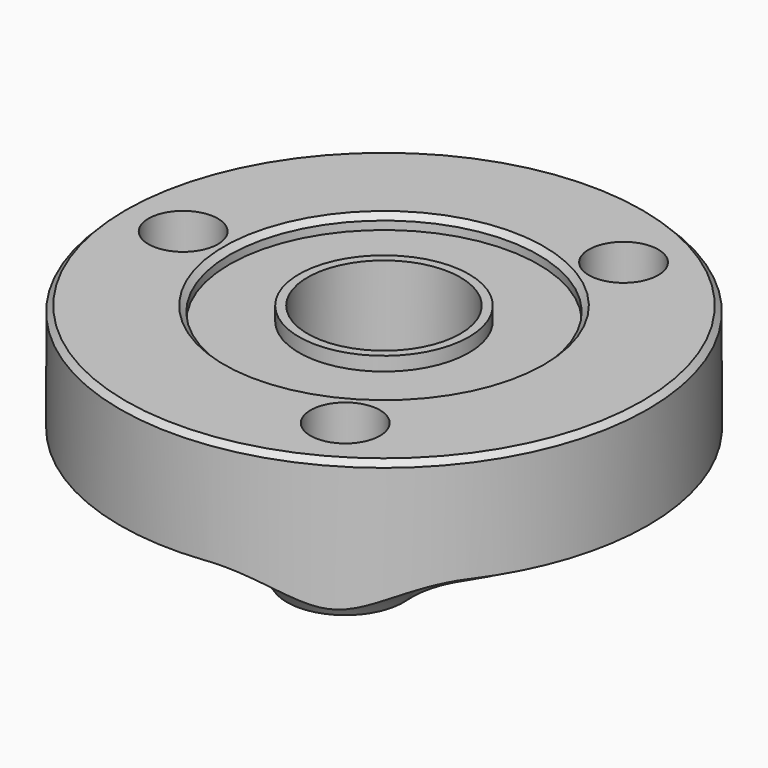
from build123d import *

# Parameters (mm, degrees)
F0_R         = 12.065
F0_R_2       = 1.5875
F0_R_3       = 3.8862
F0_R_4       = 3.4925
F1_DEPTH     = 6.35
F2_R         = 7.0612
F2_R_2       = 3.8862
F3_DEPTH     = 0.635
F4_SIZE      = 0.254
F5_R         = 12.065
F6_DEPTH     = 1.4224
F7_T2_ANGLE  = 68.0844261326
F7_T6_ANGLE  = 38.3538722805
F7_S7_R      = 12.065
F7_T8_DEPTH  = 3
F7_T12_ANGLE = 128.6233184284
F7_S13_R     = 12.065
F7_T14_DEPTH = 7
F7_T18_ANGLE = 38.3538722805
F7_S19_R     = 12.065
F7_T20_DEPTH = 3
F7_T24_ANGLE = 128.6233184284
F7_S25_R     = 12.065
F7_T26_DEPTH = 9
F7_T28_ANGLE = 68.0844261326
F7_T32_ANGLE = 38.3538722805
F7_S33_R     = 12.065
F7_T34_DEPTH = 3
F7_T38_ANGLE = 38.3538722805
F7_S39_R     = 12.065
F7_T40_DEPTH = 3
F7_T42_ANGLE = 68.0844261326
F7_T46_ANGLE = 38.3538722805
F7_S47_R     = 12.065
F7_T48_DEPTH = 4
F7_T52_ANGLE = 128.6233184284
F7_S53_R     = 12.065
F7_T54_DEPTH = 7
F7_T58_ANGLE = 38.3538722805
F7_S59_R     = 12.065
F7_T60_DEPTH = 4


# Not quite as in the source:
# - a fillet or chamfer that OpenCascade refuses, or shapes differently, is made with other operations: its cross-section is extruded or revolved along the edge and cut away or added


with BuildPart() as f1:
    # F0 (on Top) → F1 (new body)
    with BuildSketch(Plane.XY):
        Circle(F0_R)
        with Locations((4.59105, -7.9519318601)):
            Circle(F0_R_2, mode=Mode.SUBTRACT)
        with Locations((-9.1821, 0)):
            Circle(F0_R_2, mode=Mode.SUBTRACT)
        Circle(F0_R_3, mode=Mode.SUBTRACT)
        with Locations((4.59105, 7.9519318601)):
            Circle(F0_R_2, mode=Mode.SUBTRACT)
        Circle(F0_R_3)
        Circle(F0_R_4, mode=Mode.SUBTRACT)
    extrude(amount=F1_DEPTH)

    # F2 (on face) → F3 (cut)
    with BuildSketch(Plane.XY.offset(6.35)):
        Circle(F2_R)
        Circle(F2_R_2, mode=Mode.SUBTRACT)
    extrude(amount=-F3_DEPTH, mode=Mode.SUBTRACT)

    # F4
    f4_edges = [f1.edges().sort_by_distance(p)[0] for p in [
        (-7.0612, 0, 6.35),
        (-12.065, 0, 6.35),
    ]]
    chamfer(f4_edges, length=F4_SIZE)

    # F5 (on face) → F6 (cut)
    with BuildSketch(Plane(origin=(0, 0, 0), x_dir=(1, 0, 0), z_dir=(0, 0, -1))):
        Circle(F5_R)
        with BuildLine():
            ThreePointArc((0.6714307473, -9.5013054762), (-4.7625, -8.248891971), (-8.5640872851, -4.1691766541))
            ThreePointArc((-8.5640872851, -4.1691766541), (-9.3019875524, -3.1364431851), (-10.3381797291, -2.4034077182))
            ThreePointArc((-10.3381797291, -2.4034077182), (-11.8491, 0), (-10.3381797291, 2.4034077182))
            ThreePointArc((-10.3381797291, 2.4034077182), (-9.3019875524, 3.1364431851), (-8.5640872851, 4.1691766541))
            ThreePointArc((-8.5640872851, 4.1691766541), (-4.7625, 8.248891971), (0.6714307473, 9.5013054762))
            ThreePointArc((0.6714307473, 9.5013054762), (1.9347543004, 9.6239791186), (3.0876777249, 10.1548301334))
            ThreePointArc((3.0876777249, 10.1548301334), (5.92455, 10.261621612), (7.2505020042, 7.7514224152))
            ThreePointArc((7.2505020042, 7.7514224152), (7.367233252, 6.4875359336), (7.8926565378, 5.3321288221))
            ThreePointArc((7.8926565378, 5.3321288221), (9.525, 0), (7.8926565378, -5.3321288221))
            ThreePointArc((7.8926565378, -5.3321288221), (7.367233252, -6.4875359336), (7.2505020042, -7.7514224152))
            ThreePointArc((7.2505020042, -7.7514224152), (5.92455, -10.261621612), (3.0876777249, -10.1548301334))
            ThreePointArc((3.0876777249, -10.1548301334), (1.9347543004, -9.6239791186), (0.6714307473, -9.5013054762))
        make_face(mode=Mode.SUBTRACT)
    extrude(amount=-F6_DEPTH, mode=Mode.SUBTRACT)

    # F7: fillet of radius 2.794 on 11 edges, made by hand

    # F7_s1 → F7_t2 (revolve)
    with BuildSketch(Plane(origin=(0, 0, 0), x_dir=(0, 0, 1), z_dir=(-0.5598035509, -0.8286253583, 0))):
        with BuildLine():
            ThreePointArc((1.4224, -11.9591629855), (1.0407314863, -10.5495201939), (0, -9.525))
            Line((0, -9.525), (1.4224, -9.525))
            Line((1.4224, -9.525), (1.4224, -11.9591629855))
        make_face()
    revolve(axis=Axis((0, 0, 1.4224), (0, 0, 1)), revolution_arc=F7_T2_ANGLE)


with BuildPart() as f7_tool4:
    # F7_s5 → F7_t6 (revolve)
    with BuildSketch(Plane(origin=(0, 0, 0), x_dir=(0, 0, 1), z_dir=(0.5598035509, -0.8286253583, 0))):
        with BuildLine():
            ThreePointArc((1.4224, -11.9591629855), (1.0407314863, -10.5495201939), (0, -9.525))
            Line((0, -9.525), (1.4224, -9.525))
            Line((1.4224, -9.525), (1.4224, -11.9591629855))
        make_face()
    revolve(axis=Axis((11.049719153, 7.464980351, 1.4224), (0, 0, -1)), revolution_arc=F7_T6_ANGLE)

    # F7_s7 → F7_t8 (intersect, symmetric)
    with BuildSketch(Plane.XY.offset(0.7)):
        Circle(F7_S7_R)
    extrude(amount=F7_T8_DEPTH, both=True, mode=Mode.INTERSECT)


with BuildPart() as f1_1:
    add(f1.part)

    # F7_t3: union F7_tool4
    add(f7_tool4.part)


with BuildPart() as f7_tool10:
    # F7_s11 → F7_t12 (revolve)
    with BuildSketch(Plane(origin=(0.622097238, 8.2511711447, 0), x_dir=(0, 0, 1), z_dir=(-0.0751816441, -0.9971698553, 0))):
        with BuildLine():
            ThreePointArc((1.4224, -9.0813803384), (1.0407314863, -7.6717375468), (0, -6.6472173529))
            Line((0, -6.6472173529), (1.4224, -6.6472173529))
            Line((1.4224, -6.6472173529), (1.4224, -9.0813803384))
        make_face()
    revolve(axis=Axis((4.59105, 7.9519318601, 1.4224), (0, 0, 1)), revolution_arc=F7_T12_ANGLE)

    # F7_s13 → F7_t14 (intersect, symmetric)
    with BuildSketch(Plane.XY):
        Circle(F7_S13_R)
    extrude(amount=F7_T14_DEPTH, both=True, mode=Mode.INTERSECT)


with BuildPart() as f1_2:
    add(f1_1.part)

    # F7_t9: union F7_tool10
    add(f7_tool10.part)


with BuildPart() as f7_tool16:
    # F7_s17 → F7_t18 (revolve)
    with BuildSketch(Plane(origin=(0.622097238, -8.2511711447, 0), x_dir=(0, 0, 1), z_dir=(0.0751816441, -0.9971698553, 0))):
        with BuildLine():
            ThreePointArc((1.4224, -9.0813803384), (1.0407314863, -7.6717375468), (0, -6.6472173529))
            Line((0, -6.6472173529), (1.4224, -6.6472173529))
            Line((1.4224, -6.6472173529), (1.4224, -9.0813803384))
        make_face()
    revolve(axis=Axis((11.049719153, -7.464980351, 1.4224), (0, 0, -1)), revolution_arc=F7_T18_ANGLE)

    # F7_s19 → F7_t20 (intersect, symmetric)
    with BuildSketch(Plane.XY.offset(0.7)):
        Circle(F7_S19_R)
    extrude(amount=F7_T20_DEPTH, both=True, mode=Mode.INTERSECT)


with BuildPart() as f1_3:
    add(f1_2.part)

    # F7_t15: union F7_tool16
    add(f7_tool16.part)


with BuildPart() as f7_tool22:
    # F7_s23 → F7_t24 (revolve)
    with BuildSketch(Plane(origin=(6.8346752033, -4.6643375841, 0), x_dir=(0, 0, 1), z_dir=(-0.8259836045, 0.5636941414, 0))):
        with BuildLine():
            ThreePointArc((1.4224, -9.0813803384), (1.0407314863, -7.6717375468), (0, -6.6472173529))
            Line((0, -6.6472173529), (1.4224, -6.6472173529))
            Line((1.4224, -6.6472173529), (1.4224, -9.0813803384))
        make_face()
    revolve(axis=Axis((4.59105, -7.9519318601, 1.4224), (0, 0, 1)), revolution_arc=F7_T24_ANGLE)

    # F7_s25 → F7_t26 (intersect, symmetric)
    with BuildSketch(Plane.XY):
        Circle(F7_S25_R)
    extrude(amount=F7_T26_DEPTH, both=True, mode=Mode.INTERSECT)


with BuildPart() as f1_4:
    add(f1_3.part)

    # F7_t21: union F7_tool22
    add(f7_tool22.part)

    # F7_s27 → F7_t28 (revolve)
    with BuildSketch(Plane(origin=(0, 0, 0), x_dir=(0, 0, 1), z_dir=(0.997512386, -0.070491417, 0))):
        with BuildLine():
            ThreePointArc((1.4224, -11.9591629855), (1.0407314863, -10.5495201939), (0, -9.525))
            Line((0, -9.525), (1.4224, -9.525))
            Line((1.4224, -9.525), (1.4224, -11.9591629855))
        make_face()
    revolve(axis=Axis((0, 0, 1.4224), (0, 0, 1)), revolution_arc=F7_T28_ANGLE)


with BuildPart() as f7_tool30:
    # F7_s31 → F7_t32 (revolve)
    with BuildSketch(Plane(origin=(6.8346752033, 4.6643375841, 0), x_dir=(0, 0, 1), z_dir=(0.8259836045, 0.5636941414, 0))):
        with BuildLine():
            ThreePointArc((1.4224, -9.0813803384), (1.0407314863, -7.6717375468), (0, -6.6472173529))
            Line((0, -6.6472173529), (1.4224, -6.6472173529))
            Line((1.4224, -6.6472173529), (1.4224, -9.0813803384))
        make_face()
    revolve(axis=Axis((0.9400030462, 13.3018276666, 1.4224), (0, 0, -1)), revolution_arc=F7_T32_ANGLE)

    # F7_s33 → F7_t34 (intersect, symmetric)
    with BuildSketch(Plane.XY.offset(0.7)):
        Circle(F7_S33_R)
    extrude(amount=F7_T34_DEPTH, both=True, mode=Mode.INTERSECT)


with BuildPart() as f1_5:
    add(f1_4.part)

    # F7_t29: union F7_tool30
    add(f7_tool30.part)


with BuildPart() as f7_tool36:
    # F7_s37 → F7_t38 (revolve)
    with BuildSketch(Plane(origin=(0, 0, 0), x_dir=(0, 0, 1), z_dir=(-0.997512386, -0.070491417, 0))):
        with BuildLine():
            ThreePointArc((1.4224, -11.9591629855), (1.0407314863, -10.5495201939), (0, -9.525))
            Line((0, -9.525), (1.4224, -9.525))
            Line((1.4224, -9.525), (1.4224, -11.9591629855))
        make_face()
    revolve(axis=Axis((0.9400030462, -13.3018276666, 1.4224), (0, 0, -1)), revolution_arc=F7_T38_ANGLE)

    # F7_s39 → F7_t40 (intersect, symmetric)
    with BuildSketch(Plane.XY.offset(0.7)):
        Circle(F7_S39_R)
    extrude(amount=F7_T40_DEPTH, both=True, mode=Mode.INTERSECT)


with BuildPart() as f1_6:
    add(f1_5.part)

    # F7_t35: union F7_tool36
    add(f7_tool36.part)

    # F7_s41 → F7_t42 (revolve)
    with BuildSketch(Plane(origin=(0, 0, 0), x_dir=(0, 0, 1), z_dir=(-0.4377088351, 0.8991167753, 0))):
        with BuildLine():
            ThreePointArc((1.4224, -11.9591629855), (1.0407314863, -10.5495201939), (0, -9.525))
            Line((0, -9.525), (1.4224, -9.525))
            Line((1.4224, -9.525), (1.4224, -11.9591629855))
        make_face()
    revolve(axis=Axis((0, 0, 1.4224), (0, 0, 1)), revolution_arc=F7_T42_ANGLE)


with BuildPart() as f7_tool44:
    # F7_s45 → F7_t46 (revolve)
    with BuildSketch(Plane(origin=(0, 0, 0), x_dir=(0, 0, 1), z_dir=(0.4377088351, 0.8991167753, 0))):
        with BuildLine():
            ThreePointArc((1.4224, -11.9591629855), (1.0407314863, -10.5495201939), (0, -9.525))
            Line((0, -9.525), (1.4224, -9.525))
            Line((1.4224, -9.525), (1.4224, -11.9591629855))
        make_face()
    revolve(axis=Axis((-11.9897221992, 5.8368473157, 1.4224), (0, 0, -1)), revolution_arc=F7_T46_ANGLE)

    # F7_s47 → F7_t48 (intersect, symmetric)
    with BuildSketch(Plane.XY.offset(0.7)):
        Circle(F7_S47_R)
    extrude(amount=F7_T48_DEPTH, both=True, mode=Mode.INTERSECT)


with BuildPart() as f1_7:
    add(f1_6.part)

    # F7_t43: union F7_tool44
    add(f7_tool44.part)


with BuildPart() as f7_tool50:
    # F7_s51 → F7_t52 (revolve)
    with BuildSketch(Plane(origin=(-7.4567724413, -3.5868335607, 0), x_dir=(0, 0, 1), z_dir=(0.9011652487, 0.4334757139, 0))):
        with BuildLine():
            ThreePointArc((1.4224, -9.0813803384), (1.0407314863, -7.6717375468), (0, -6.6472173529))
            Line((0, -6.6472173529), (1.4224, -6.6472173529))
            Line((1.4224, -6.6472173529), (1.4224, -9.0813803384))
        make_face()
    revolve(axis=Axis((-9.1821, 0, 1.4224), (0, 0, 1)), revolution_arc=F7_T52_ANGLE)

    # F7_s53 → F7_t54 (intersect, symmetric)
    with BuildSketch(Plane.XY):
        Circle(F7_S53_R)
    extrude(amount=F7_T54_DEPTH, both=True, mode=Mode.INTERSECT)


with BuildPart() as f1_8:
    add(f1_7.part)

    # F7_t49: union F7_tool50
    add(f7_tool50.part)


with BuildPart() as f7_tool56:
    # F7_s57 → F7_t58 (revolve)
    with BuildSketch(Plane(origin=(-7.4567724413, 3.5868335607, 0), x_dir=(0, 0, 1), z_dir=(-0.9011652487, 0.4334757139, 0))):
        with BuildLine():
            ThreePointArc((1.4224, -9.0813803384), (1.0407314863, -7.6717375468), (0, -6.6472173529))
            Line((0, -6.6472173529), (1.4224, -6.6472173529))
            Line((1.4224, -6.6472173529), (1.4224, -9.0813803384))
        make_face()
    revolve(axis=Axis((-11.9897221992, -5.8368473157, 1.4224), (0, 0, -1)), revolution_arc=F7_T58_ANGLE)

    # F7_s59 → F7_t60 (intersect, symmetric)
    with BuildSketch(Plane.XY.offset(0.7)):
        Circle(F7_S59_R)
    extrude(amount=F7_T60_DEPTH, both=True, mode=Mode.INTERSECT)


with BuildPart() as f1_9:
    add(f1_8.part)

    # F7_t55: union F7_tool56
    add(f7_tool56.part)


solid = f1_9.part
